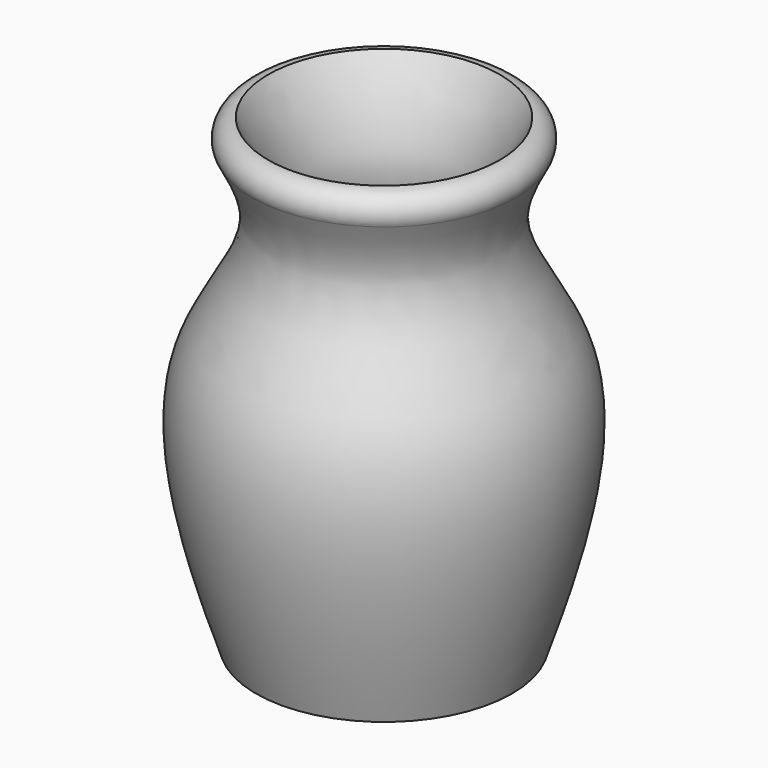
from build123d import *

# Parameters (mm, degrees)
F2_T = -3


# Not quite as in the source:
# - a fillet or chamfer that OpenCascade refuses, or shapes differently, is made with other operations: its cross-section is extruded or revolved along the edge and cut away or added


with BuildPart() as f1:
    # F0 (on Front) → F1 (revolve)
    with BuildSketch(Plane.XZ):
        with BuildLine():
            add(Edge.make_bspline(
                [(15.8777516335, 49.7320406139), (13.74524129, 46.2605530647), (9.2830394347, 38.9965891498), (19.8781052941, 27.7064520444), (17.5417256826, 11.5760115727), (14.9212029016, 3.7049304204), (13.6877186596, 0)],
                knots=[0, 0, 0, 0, 0.2310726214, 0.483511221, 0.7568879101, 1, 1, 1, 1], degree=3))
            Line((15.8777516335, 49.7320406139), (0, 49.7320406139))
            Line((0, 49.7320406139), (0, 0))
            Line((0, 0), (13.6877186596, 0))
        make_face()
    revolve(axis=Axis((0, 0, 26.1985007674), (0, 0, 1)))

    # F2
    f2_openings = [f1.faces().sort_by_distance(p)[0] for p in [
        (0, 0, 49.732041),
    ]]
    offset(amount=F2_T, openings=f2_openings)

    # F3: fillet of radius 2 on 1 edges, made by hand

    # F3_s1 → F3_t2 (revolve, cut)
    with BuildSketch(Plane.XZ):
        with BuildLine():
            ThreePointArc((14.1128151685, 46.7623575212), (14.0873533023, 48.7462971371), (12.3654431699, 49.7320406139))
            Line((12.3654431699, 49.7320406139), (12.365479801, 49.7720405971))
            Line((12.365479801, 49.7720405971), (15.8777516335, 49.7720406139))
            Line((15.8777516335, 49.7720406139), (15.9118345629, 49.7111037105))
            ThreePointArc((15.9118345629, 49.7111037105), (15.013225293, 48.236442696), (14.1477992396, 46.7429638426))
            Line((14.1477992396, 46.7429638426), (14.1128151685, 46.7623575212))
        make_face()
    revolve(axis=Axis((0, 0, 49.7320406139), (0, 0, 1)), mode=Mode.SUBTRACT)


solid = f1.part
